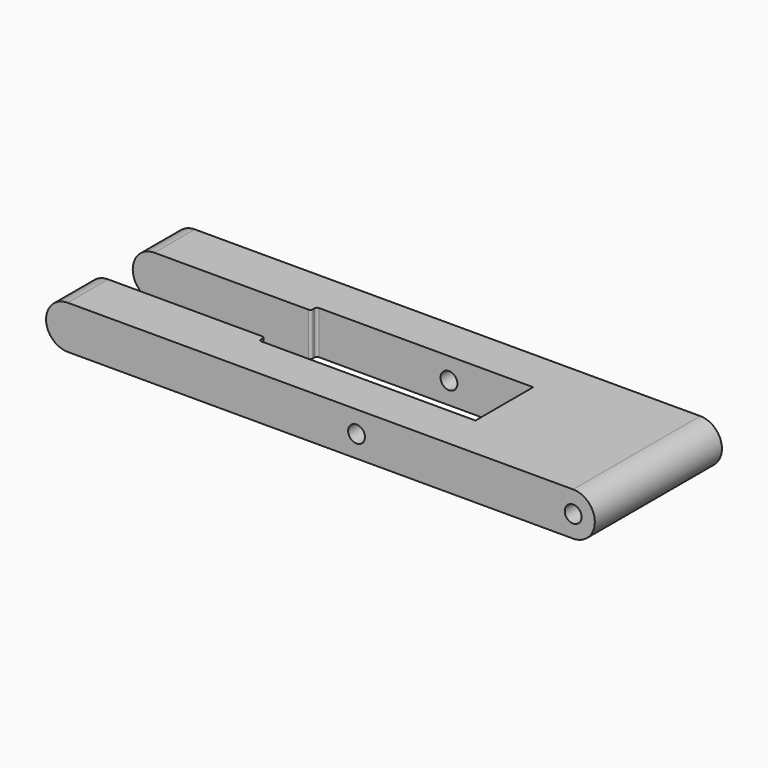
from build123d import *

# Parameters (mm, degrees)
F1_DEPTH    = 16.5
F3_D        = 3.5
F4_W        = 40
F4_H        = 12
F5_DEPTH    = 25
F7_T1_DEPTH = 15
F8_R        = 0.5


# Not quite as in the source:
# - a fillet or chamfer that OpenCascade refuses, or shapes differently, is made with other operations: its cross-section is extruded or revolved along the edge and cut away or added


with BuildPart() as f1:
    # F0 (on Front) → F1 (new body, symmetric)
    with BuildSketch(Plane.XZ):
        with BuildLine():
            ThreePointArc((-52.5, 9), (-57, 4.5), (-52.5, 0))
            Line((-52.5, 0), (52.5, 0))
            ThreePointArc((52.5, 0), (57, 4.5), (52.5, 9))
            Line((52.5, 9), (-52.5, 9))
        make_face()
    extrude(amount=F1_DEPTH, both=True)

    # F3 (through all)
    with Locations(Plane.XZ.offset(16.5)):
        with Locations((7.5, 4.5), (52.5, 4.5)):
            Hole(F3_D / 2)


with BuildPart() as f5:
    # F4 (on Top) → F5 (new body)
    with BuildSketch(Plane.XY):
        Polygon((15, 7.5), (-20, 7.5), (-20, 6), (-20, -6), (-20, -7.5), (15, -7.5), align=None)
        with Locations((-40, 0)):
            Rectangle(F4_W, F4_H)
    extrude(amount=F5_DEPTH)


with BuildPart() as f1_1:
    add(f1.part)

    # F6: cut F5
    add(f5.part, mode=Mode.SUBTRACT)

    # F7: chamfer of 10 on 1 edges, made by hand

    # F7_s2 → F7_t1 (cut)
    with BuildSketch(Plane.XZ.offset(-7.5)):
        with BuildLine():
            Line((25.2828427125, 9.2828427125), (14.7171572875, -1.2828427125))
            Line((14.7171572875, -1.2828427125), (14.5171572875, -1.2828427125))
            ThreePointArc((14.5171572875, -1.2828427125), (14.8, 3.8585786438), (14.8, 9))
            Line((14.8, 9), (15, 9.2))
            ThreePointArc((15, 9.2), (20.1414213562, 9.2), (25.2828427125, 9.4828427125))
            Line((25.2828427125, 9.4828427125), (25.2828427125, 9.2828427125))
        make_face()
    extrude(amount=F7_T1_DEPTH, mode=Mode.SUBTRACT)

    # F8
    f8_edges = [f1_1.edges().sort_by_distance(p)[0] for p in [
        (-20, 7.5, 4.5),
        (-20, 6, 4.5),
        (-20, -7.5, 4.5),
        (-20, -6, 4.5),
    ]]
    fillet(f8_edges, radius=F8_R)


solid = f1_1.part
